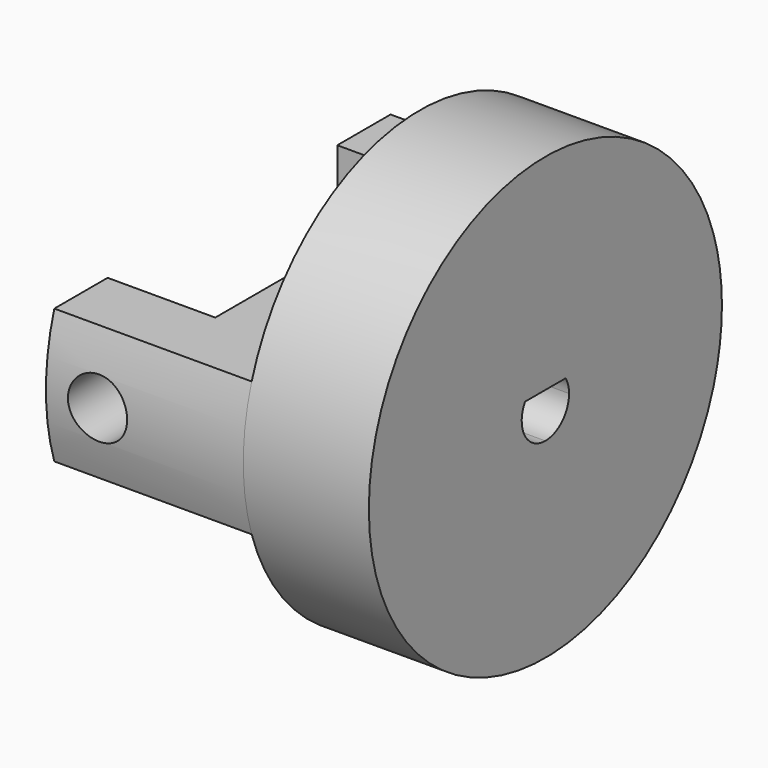
from build123d import *
from build123d import SkipClean  # not in build123d's __all__

# Parameters (mm, degrees)
F1_DEPTH = 7.5
F3_DEPTH = 25.001
F5_DEPTH = 7
F7_DEPTH = 25
F8_R     = 14.6869623893
F8_R_2   = 12.3
F9_DEPTH = 25


with BuildPart() as f1:
    # F0 (on Top) → F1 (new body)
    with BuildSketch(Plane.XY):
        Polygon((5.5, -12.5), (5.5, 12.5), (-5.5, 12.5), (-5.5, 8), (0.5, 8), (0.5, -8), (-5.5, -8), (-5.5, -12.5), align=None)
    extrude(amount=F1_DEPTH)

    # F2 (on face) → F3 (cut, through all)
    with BuildSketch(Plane(origin=(0, 12.5, 0), x_dir=(-1, 0, 0), z_dir=(0, 1, 0))):
        with BuildLine():
            ThreePointArc((4.273, 3.75), (2.623, 5.4), (0.973, 3.75))
            Line((0.973, 3.75), (4.273, 3.75))
        make_face()
        with BuildLine():
            Line((4.273, 3.75), (0.973, 3.75))
            ThreePointArc((0.973, 3.75), (2.623, 2.1), (4.273, 3.75))
        make_face()
    extrude(amount=-F3_DEPTH, mode=Mode.SUBTRACT)

    # F4 (on face) → F5 (join)
    with BuildSketch(Plane.YZ.offset(5.5)):
        with BuildLine():
            Line((-11.7144141979, 7.5), (0, 7.5))
            Line((0, 7.5), (11.7144141979, 7.5))
            ThreePointArc((11.7144141979, 7.5), (0, 16.05), (-11.7144141979, 7.5))
        make_face()
        with BuildLine():
            Line((0, 0), (0, 7.5))
            Line((0, 7.5), (-11.7144141979, 7.5))
            ThreePointArc((-11.7144141979, 7.5), (-12.3, 3.75), (-11.7144141979, 0))
            Line((-11.7144141979, 0), (0, 0))
        make_face()
        with BuildLine():
            Line((11.7144141979, 0), (0, 0))
            Line((0, 0), (-11.7144141979, 0))
            ThreePointArc((-11.7144141979, 0), (0, -8.55), (11.7144141979, 0))
        make_face()
        with BuildLine():
            Line((11.7144141979, 7.5), (0, 7.5))
            Line((0, 7.5), (0, 0))
            Line((0, 0), (11.7144141979, 0))
            ThreePointArc((11.7144141979, 0), (12.1527218069, 1.8522769741), (12.3, 3.75))
            ThreePointArc((12.3, 3.75), (12.1527218069, 5.6477230259), (11.7144141979, 7.5))
        make_face()
    extrude(amount=F5_DEPTH)

    # F6 (on face) → F7 (cut)
    with BuildSketch(Plane.YZ.offset(12.5)):
        with BuildLine():
            Line((0, 2.1), (0, 4.6))
            Line((0, 4.6), (-1.4142135624, 4.6))
            ThreePointArc((-1.4142135624, 4.6), (-1.4361406616, 2.9375961595), (0, 2.1))
        make_face()
        with BuildLine():
            Line((1.4142135624, 4.6), (0, 4.6))
            Line((0, 4.6), (0, 2.1))
            ThreePointArc((0, 2.1), (1.166726189, 2.583273811), (1.65, 3.75))
            ThreePointArc((1.65, 3.75), (1.5899610652, 4.1910485359), (1.4142135624, 4.6))
        make_face()
    extrude(amount=-F7_DEPTH, mode=Mode.SUBTRACT)

    # F8 (on face) → F9 (cut)
    with BuildSketch(Plane.YZ.offset(12.5)):
        with Locations((0, 3.75)):
            Circle(F8_R)
        with Locations((0, 3.75)):
            Circle(F8_R_2, mode=Mode.SUBTRACT)
    with SkipClean():  # cleaning this boolean's faces spoils the solid; the shape is the same uncleaned
        extrude(amount=-F9_DEPTH, mode=Mode.SUBTRACT)


solid = f1.part
